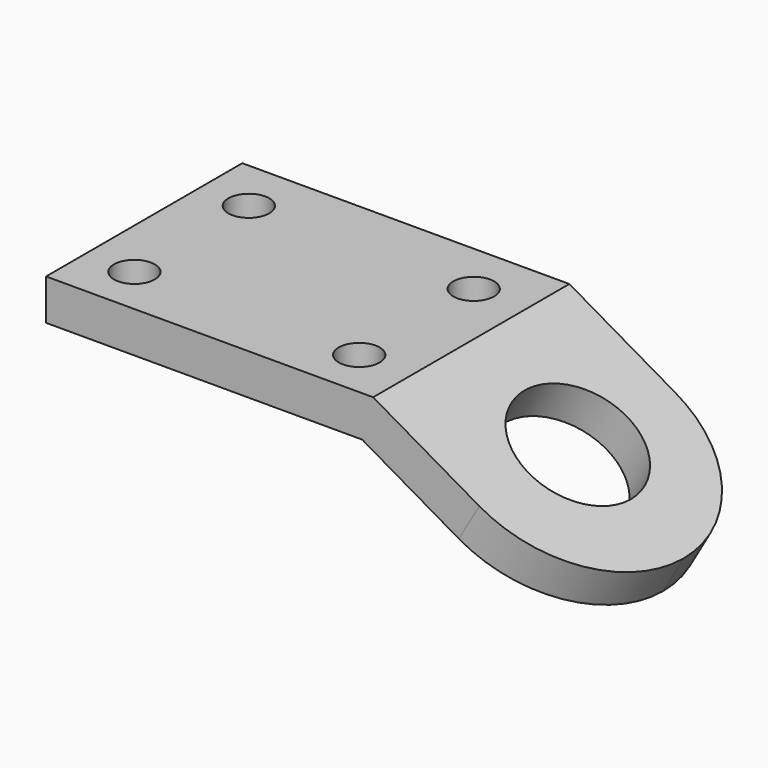
from build123d import *

# Parameters (mm, degrees)
F1_DEPTH = 60
F2_R     = 29.99999
F3_R     = 15
F4_DEPTH = 78.3
F5_R     = 5
F6_DEPTH = 25


# Not quite as in the source:
# - a fillet or chamfer is up to 0.001 mm smaller than in the source, because OpenCascade refuses the exact size


with BuildPart() as f1:
    # F0 (on Front) → F1 (new body)
    with BuildSketch(Plane.XZ):
        Polygon((80, 0), (0, 0), (0, -10), (77.3205080757, -10), (126.9615242271, -38.6602540378), (131.9615242271, -30), align=None)
    extrude(amount=-F1_DEPTH)

    # F2 (radius 30 in the source; OpenCascade refuses exactly that, so slightly less here)
    f2_edges = [f1.edges().sort_by_distance(p)[0] for p in [
        (129.461524, 60, -34.330127),
        (129.461524, 0, -34.330127),
    ]]
    fillet(f2_edges, radius=F2_R)

    # F3 (on face) → F4 (cut)
    with BuildSketch(Plane(origin=(20, 0, 34.6410161514), x_dir=(0.8660254038, 0, -0.5), z_dir=(0.5, 0, 0.8660254038))):
        with Locations((98.4833240509, 30.9668332338)):
            Circle(F3_R)
    extrude(amount=-F4_DEPTH, mode=Mode.SUBTRACT)

    # F5 (on face) → F6 (cut)
    with BuildSketch(Plane.XY):
        with Locations((12, 47)):
            Circle(F5_R)
        with Locations((12, 12)):
            Circle(F5_R)
        with Locations((67, 12)):
            Circle(F5_R)
        with Locations((67, 47)):
            Circle(F5_R)
    extrude(amount=-F6_DEPTH, mode=Mode.SUBTRACT)


solid = f1.part
